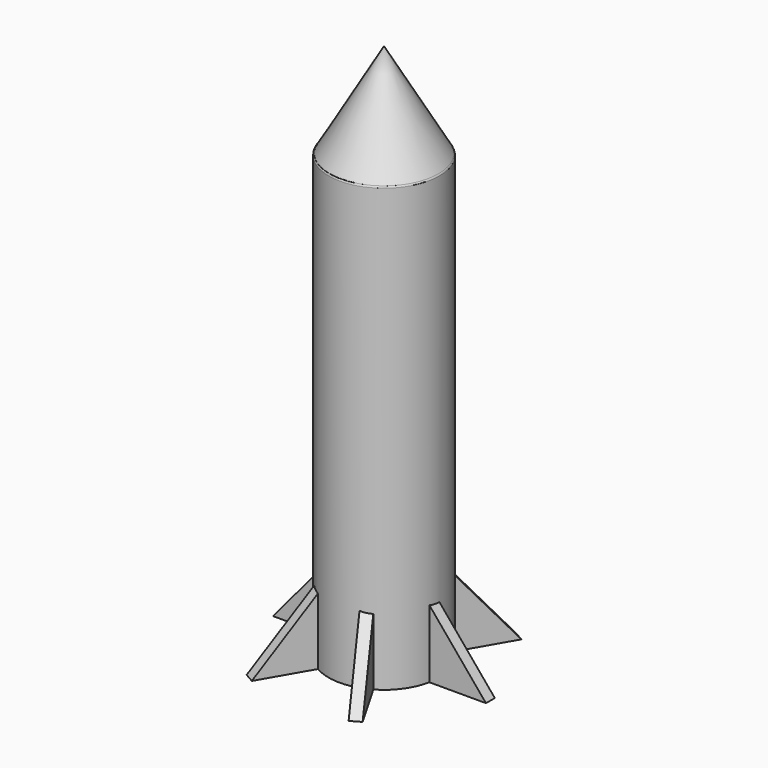
from build123d import *

# Parameters (mm, degrees)
F0_R            = 125
F1_DEPTH        = 1000
F6_DEPTH        = 25
F6_COPIES_COUNT = 6


# Not quite as in the source:
# - a fillet or chamfer that OpenCascade refuses, or shapes differently, is made with other operations: its cross-section is extruded or revolved along the edge and cut away or added
# - a pattern or mirror of a feature is missing from the dataset's text; its kind, count and spacing are read off the source's solid


with BuildPart() as f1:
    # F0 (on Top) → F1 (new body)
    with BuildSketch(Plane.XY):
        Circle(F0_R)
    extrude(amount=F1_DEPTH)

    # F2 (on Front) → F3 (revolve)
    with BuildSketch(Plane.XZ):
        Polygon((-124.5536804199, 997.6518154144), (0, 998.6120462418), (0, 1213.404417038), align=None)
    revolve(axis=Axis((0, 0, 1106.0082316399), (0, 0, 1)))

    # F4: fillet of radius 5 on 1 edges, made by hand

    # F4_s1 → F4_t2 (revolve, cut)
    with BuildSketch(Plane.XZ):
        with BuildLine():
            ThreePointArc((125, 996.1565242927), (124.5271615516, 998.2789776575), (123.1980766857, 1000))
            Line((123.1980766857, 1000), (125, 1000))
            Line((125, 1000), (125, 996.1565242927))
        make_face()
    revolve(axis=Axis((0, 0, 1000), (0, 0, 1)), mode=Mode.SUBTRACT)

    # F5 (on Front) → F6 (join)
    with BuildSketch(Plane.XZ):
        Polygon((0, 300), (0, 0), (250, 0), align=None)
    f6 = extrude(amount=F6_DEPTH)

    # F6_copies: F6 ×6 about axis
    f6_copies_axis = Axis((0, 0, 0), (0, 0, 1))
    for i in range(1, F6_COPIES_COUNT):
        add(f6.rotate(f6_copies_axis, i * 360 / F6_COPIES_COUNT))


solid = f1.part
